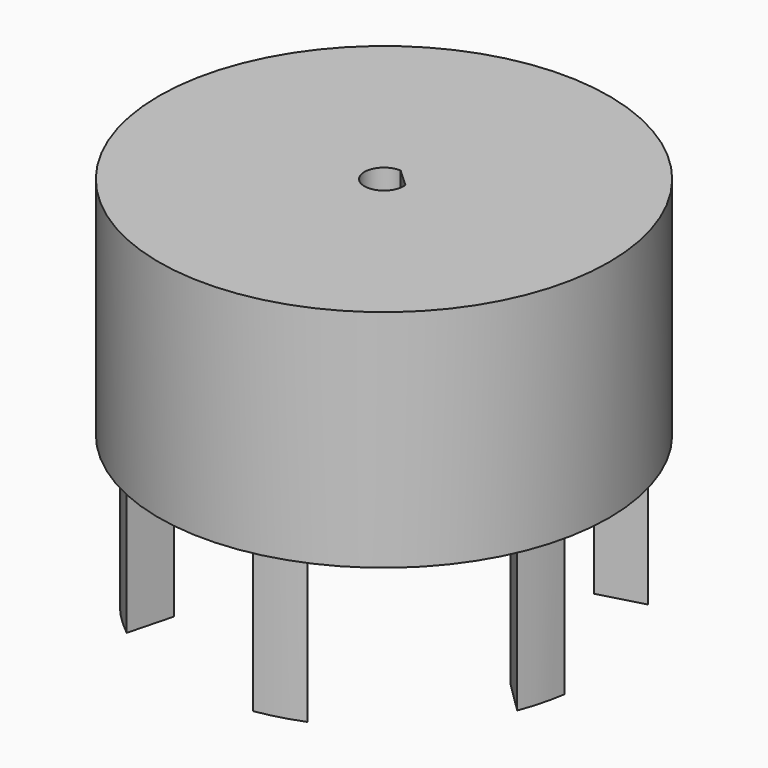
from build123d import *

# Parameters (mm, degrees)
F1_R     = 30
F2_DEPTH = 10
F5_DEPTH = 40
F3_R     = 30
F3_R_2   = 27.5
F6_DEPTH = 20


with BuildPart() as f2:
    # F1 (on face) → F2 (new body)
    with BuildSketch(Plane.XY):
        Circle(F1_R)
        with BuildLine():
            ThreePointArc((2.6, 0), (-1.8887723072, -1.7867678001), (0.1442006372, 2.5959981079))
            Line((0.1442006372, 2.5959981079), (1.3613009588, 1.465216605))
            Line((1.3613009588, 1.465216605), (2.5784012803, 0.3344351021))
            ThreePointArc((2.5784012803, 0.3344351021), (2.5945947014, 0.1675659141), (2.6, 0))
        make_face(mode=Mode.SUBTRACT)
    extrude(amount=F2_DEPTH)

    # F4 (on face) → F5 (join)
    with BuildSketch(Plane(origin=(0, 0, 0), x_dir=(1, 0, 0), z_dir=(0, 0, -1))):
        with BuildLine():
            Line((25.6627975095, 9.8828550524), (21.2857162159, 5.5604213128))
            Line((21.2857162159, 5.5604213128), (27.2175942873, 3.9309745879))
            ThreePointArc((27.2175942873, 3.9309745879), (26.6071452699, 6.950526641), (25.6627975095, 9.8828550524))
        make_face()
        with BuildLine():
            Line((21.390202292, -17.2832070492), (15.4583242206, -15.6537603243))
            Line((15.4583242206, -15.6537603243), (17.0131209984, -21.6056407888))
            ThreePointArc((17.0131209984, -21.6056407888), (19.3229052758, -19.5672004054), (21.390202292, -17.2832070492))
        make_face()
        with BuildLine():
            Line((4.2725952175, 27.1660621016), (5.8273919953, 21.2141816371))
            Line((5.8273919953, 21.2141816371), (10.2044732889, 25.5366153767))
            ThreePointArc((10.2044732889, 25.5366153767), (7.2842399941, 26.5177270464), (4.2725952175, 27.1660621016))
        make_face()
        with BuildLine():
            Line((-4.2725952175, -27.1660621016), (-5.8273919953, -21.2141816371))
            Line((-5.8273919953, -21.2141816371), (-10.2044732889, -25.5366153767))
            ThreePointArc((-10.2044732889, -25.5366153767), (-7.2842399941, -26.5177270464), (-4.2725952175, -27.1660621016))
        make_face()
        with BuildLine():
            Line((-21.390202292, 17.2832070492), (-15.4583242206, 15.6537603243))
            Line((-15.4583242206, 15.6537603243), (-17.0131209984, 21.6056407888))
            ThreePointArc((-17.0131209984, 21.6056407888), (-19.3229052758, 19.5672004054), (-21.390202292, 17.2832070492))
        make_face()
        with BuildLine():
            Line((-25.6627975095, -9.8828550524), (-21.2857162159, -5.5604213128))
            Line((-21.2857162159, -5.5604213128), (-27.2175942873, -3.9309745879))
            ThreePointArc((-27.2175942873, -3.9309745879), (-26.6071452699, -6.950526641), (-25.6627975095, -9.8828550524))
        make_face()
    extrude(amount=F5_DEPTH)

    # F3 (on face) → F6 (join)
    with BuildSketch(Plane(origin=(0, 0, 0), x_dir=(1, 0, 0), z_dir=(0, 0, -1))):
        Circle(F3_R)
        Circle(F3_R_2, mode=Mode.SUBTRACT)
    extrude(amount=F6_DEPTH)


solid = f2.part
